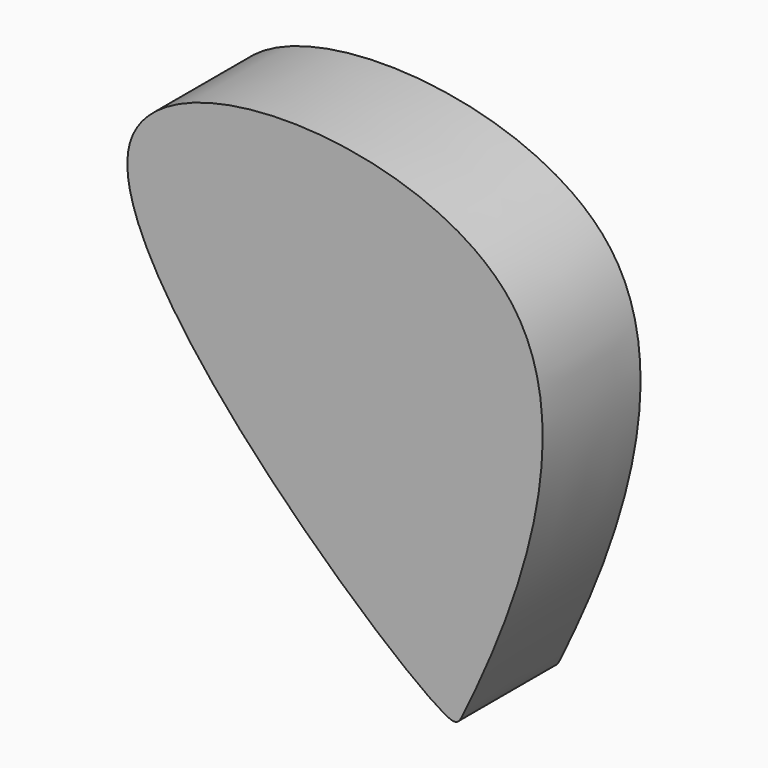
from build123d import *

# Parameters (mm, degrees)
F1_DEPTH = 25.4


with BuildPart() as f1:
    # F0 (on Front) → F1 (new body)
    with BuildSketch(Plane.XZ):
        with BuildLine():
            add(Edge.make_bspline(
                [(-40.0487333536, 44.3783216178), (-46.7732862538, 20.4935793212), (26.3876980647, -43.7381694328), (29.6041718107, -36.1805486976), (77.7443001231, 62.5175239307), (-34.2323295474, 65.0374357723), (-40.0487333536, 44.3783216178)],
                knots=[0, 0, 0, 0, 0.341076819, 0.4118937738, 0.7049855154, 1, 1, 1, 1], degree=3))
        make_face()
    extrude(amount=F1_DEPTH)


solid = f1.part
